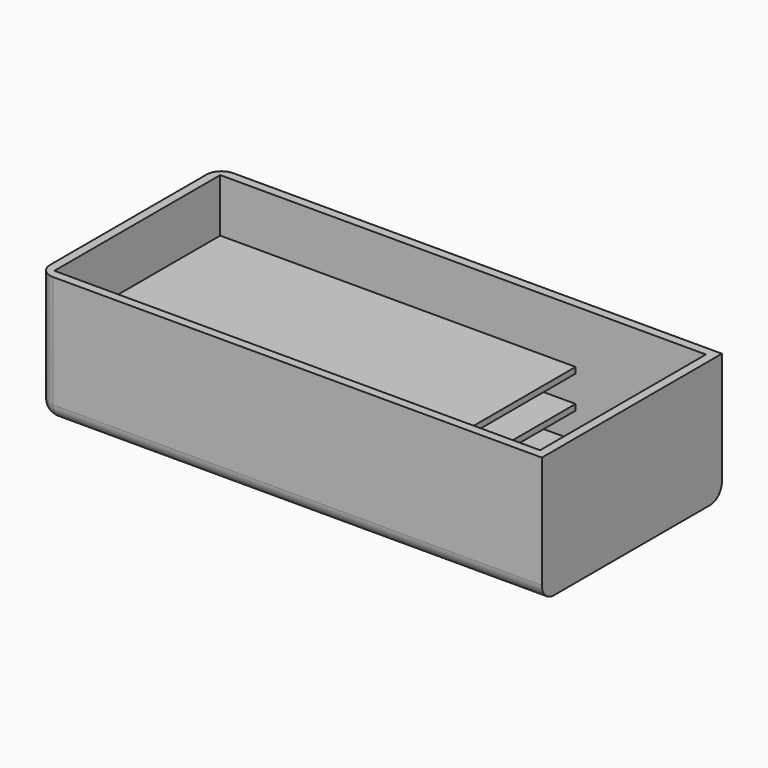
from build123d import *

# Parameters (mm, degrees)
F0_W      = 170
F0_H      = 76
F0_W_2    = 164
F0_H_2    = 70
F1_DEPTH  = 3
F2_DEPTH  = 40
F4_DEPTH  = 35.9
F5_DEPTH  = 36.4
F6_R      = 1.4
F7_DEPTH  = 0.5
F9_R      = 1.4
F10_DEPTH = 0.5
F12_R     = 5
F13_W     = 5
F13_H     = 60
F14_DEPTH = 5
F15_R     = 1


# Not quite as in the source:
# - a fillet or chamfer that OpenCascade refuses, or shapes differently, is made with other operations: its cross-section is extruded or revolved along the edge and cut away or added


with BuildPart() as f1:
    # F0 (on Top) → F1 (new body)
    with BuildSketch(Plane.XY):
        Rectangle(F0_W, F0_H)
        Rectangle(F0_W_2, F0_H_2, mode=Mode.SUBTRACT)
        Rectangle(F0_W_2, F0_H_2)
    extrude(amount=-F1_DEPTH)

    # F0 (on Top) → F2 (join)
    with BuildSketch(Plane.XY):
        Rectangle(F0_W, F0_H)
        Rectangle(F0_W_2, F0_H_2, mode=Mode.SUBTRACT)
    extrude(amount=F2_DEPTH)

    # F3 (on Front) → F4 (join, symmetric)
    with BuildSketch(Plane.XZ):
        Polygon((-82, 11), (-82, 9), (-71, 9), (0, 9), (5.6, 9), (38, 9), (38, 11), align=None)
    extrude(amount=F4_DEPTH, both=True)

    # F3 (on Front) → F5 (join, symmetric)
    with BuildSketch(Plane.XZ):
        Polygon((-82, 22), (-82, 20), (-71, 20), (5.6, 20), (38, 20), (38, 22), align=None)
    extrude(amount=F5_DEPTH, both=True)

    # F6 (on face) → F7 (join)
    with BuildSketch(Plane.XZ.offset(-35)):
        with Locations((-71, 16)):
            Circle(F6_R)
        with Locations((-71, 5)):
            Circle(F6_R)
        with Locations((5.6, 5)):
            Circle(F6_R)
        with Locations((5.6, 16)):
            Circle(F6_R)
    extrude(amount=F7_DEPTH)

    # F8: fillet of radius 1 on 4 edges, made by hand

    # F8_s1 → F8_t2 (revolve, cut)
    with BuildSketch(Plane.XY.offset(16)):
        with BuildLine():
            ThreePointArc((-69.6, 35), (-69.9660254038, 34.6339745962), (-70.4660254038, 34.5))
            Line((-70.4660254038, 34.5), (-69.6, 34.5))
            Line((-69.6, 34.5), (-69.6, 35))
        make_face()
    revolve(axis=Axis((-71, 34.5, 16), (0, -1, 0)), mode=Mode.SUBTRACT)

    # F8_s3 → F8_t4 (revolve, cut)
    with BuildSketch(Plane.XY.offset(5)):
        with BuildLine():
            ThreePointArc((-69.6, 35), (-69.9660254038, 34.6339745962), (-70.4660254038, 34.5))
            Line((-70.4660254038, 34.5), (-69.6, 34.5))
            Line((-69.6, 34.5), (-69.6, 35))
        make_face()
    revolve(axis=Axis((-71, 34.5, 5), (0, -1, 0)), mode=Mode.SUBTRACT)

    # F8_s5 → F8_t6 (revolve, cut)
    with BuildSketch(Plane.XY.offset(16)):
        with BuildLine():
            ThreePointArc((7, 35), (6.6339745962, 34.6339745962), (6.1339745962, 34.5))
            Line((6.1339745962, 34.5), (7, 34.5))
            Line((7, 34.5), (7, 35))
        make_face()
    revolve(axis=Axis((5.6, 34.5, 16), (0, -1, 0)), mode=Mode.SUBTRACT)

    # F8_s7 → F8_t8 (revolve, cut)
    with BuildSketch(Plane.XY.offset(5)):
        with BuildLine():
            ThreePointArc((7, 35), (6.6339745962, 34.6339745962), (6.1339745962, 34.5))
            Line((6.1339745962, 34.5), (7, 34.5))
            Line((7, 34.5), (7, 35))
        make_face()
    revolve(axis=Axis((5.6, 34.5, 5), (0, -1, 0)), mode=Mode.SUBTRACT)

    # F9 (on face) → F10 (join)
    with BuildSketch(Plane(origin=(0, -35, 0), x_dir=(-1, 0, 0), z_dir=(0, 1, 0))):
        with Locations((71, 16)):
            Circle(F9_R)
        with Locations((-5.6, 16)):
            Circle(F9_R)
        with Locations((-5.6, 5)):
            Circle(F9_R)
        with Locations((71, 5)):
            Circle(F9_R)
    extrude(amount=F10_DEPTH)

    # F11: fillet of radius 1 on 4 edges, made by hand

    # F11_s1 → F11_t2 (revolve, cut)
    with BuildSketch(Plane.XY.offset(16)):
        with BuildLine():
            ThreePointArc((-72.4, -35), (-72.0339745962, -34.6339745962), (-71.5339745962, -34.5))
            Line((-71.5339745962, -34.5), (-72.4, -34.5))
            Line((-72.4, -34.5), (-72.4, -35))
        make_face()
    revolve(axis=Axis((-71, -34.5, 16), (0, 1, 0)), mode=Mode.SUBTRACT)

    # F11_s3 → F11_t4 (revolve, cut)
    with BuildSketch(Plane.XY.offset(5)):
        with BuildLine():
            ThreePointArc((-72.4, -35), (-72.0339745962, -34.6339745962), (-71.5339745962, -34.5))
            Line((-71.5339745962, -34.5), (-72.4, -34.5))
            Line((-72.4, -34.5), (-72.4, -35))
        make_face()
    revolve(axis=Axis((-71, -34.5, 5), (0, 1, 0)), mode=Mode.SUBTRACT)

    # F11_s5 → F11_t6 (revolve, cut)
    with BuildSketch(Plane.XY.offset(16)):
        with BuildLine():
            ThreePointArc((4.2, -35), (4.5660254038, -34.6339745962), (5.0660254038, -34.5))
            Line((5.0660254038, -34.5), (4.2, -34.5))
            Line((4.2, -34.5), (4.2, -35))
        make_face()
    revolve(axis=Axis((5.6, -34.5, 16), (0, 1, 0)), mode=Mode.SUBTRACT)

    # F11_s7 → F11_t8 (revolve, cut)
    with BuildSketch(Plane.XY.offset(5)):
        with BuildLine():
            ThreePointArc((4.2, -35), (4.5660254038, -34.6339745962), (5.0660254038, -34.5))
            Line((5.0660254038, -34.5), (4.2, -34.5))
            Line((4.2, -34.5), (4.2, -35))
        make_face()
    revolve(axis=Axis((5.6, -34.5, 5), (0, 1, 0)), mode=Mode.SUBTRACT)

    # F12
    f12_edges = [f1.edges().sort_by_distance(p)[0] for p in [
        (-85, 38, 18.5),
        (-85, -38, 18.5),
        (-85, 0, -3),
        (0, 38, -3),
        (0, -38, -3),
    ]]
    fillet(f12_edges, radius=F12_R)

    # F13 (on face) → F14 (cut)
    with BuildSketch(Plane.XY):
        Rectangle(F13_W, F13_H)
    extrude(amount=-F14_DEPTH, mode=Mode.SUBTRACT)

    # F15
    f15_edges = [f1.edges().sort_by_distance(p)[0] for p in [
        (0, 30, 0),
        (-2.5, 30, -1.5),
        (0, 30, -3),
        (2.5, 30, -1.5),
        (0, -30, 0),
        (2.5, -30, -1.5),
        (0, -30, -3),
        (-2.5, -30, -1.5),
        (-2.5, 0, -3),
        (2.5, 0, -3),
        (-2.5, 0, 0),
        (2.5, 0, 0),
    ]]
    fillet(f15_edges, radius=F15_R)


solid = f1.part
